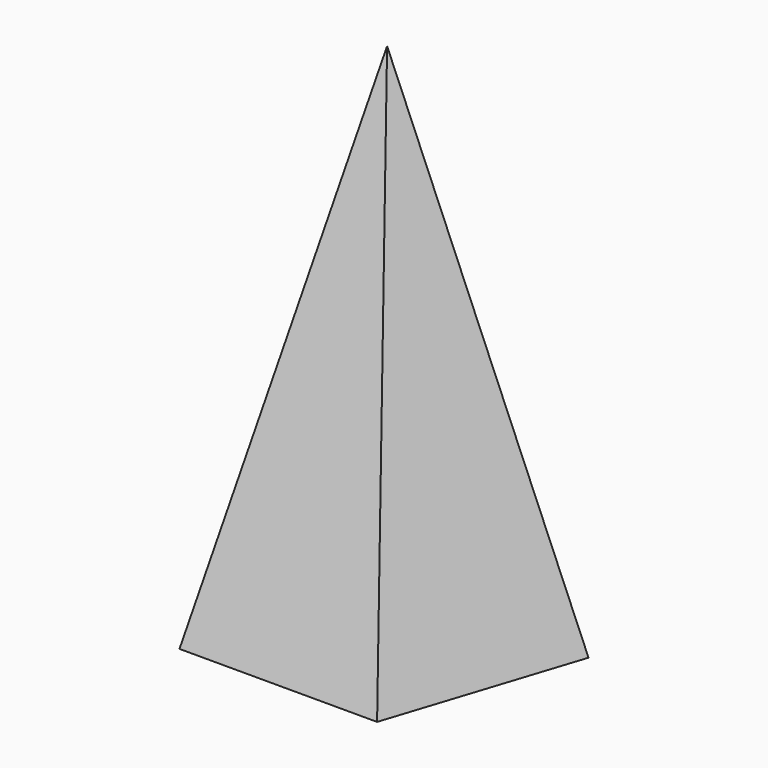
from build123d import *


# Not quite as in the source:
# - an extrude whose draft closes it to a point is written as a loft to that point


with BuildPart() as f1:
    # F0 (on Top) → F1 section 0
    with BuildSketch(Plane.XY, mode=Mode.PRIVATE) as f1_s0:
        Polygon((13.9262220778, -19.1678002884), (22.5331006568, 7.3214482206), (0, 23.6927041356), (-22.5331006568, 7.3214482206), (-13.9262220778, -19.1678002884), align=None)
    loft([f1_s0.sketch, Vertex(0, 0, 71.5352045456)], ruled=True)


solid = f1.part
